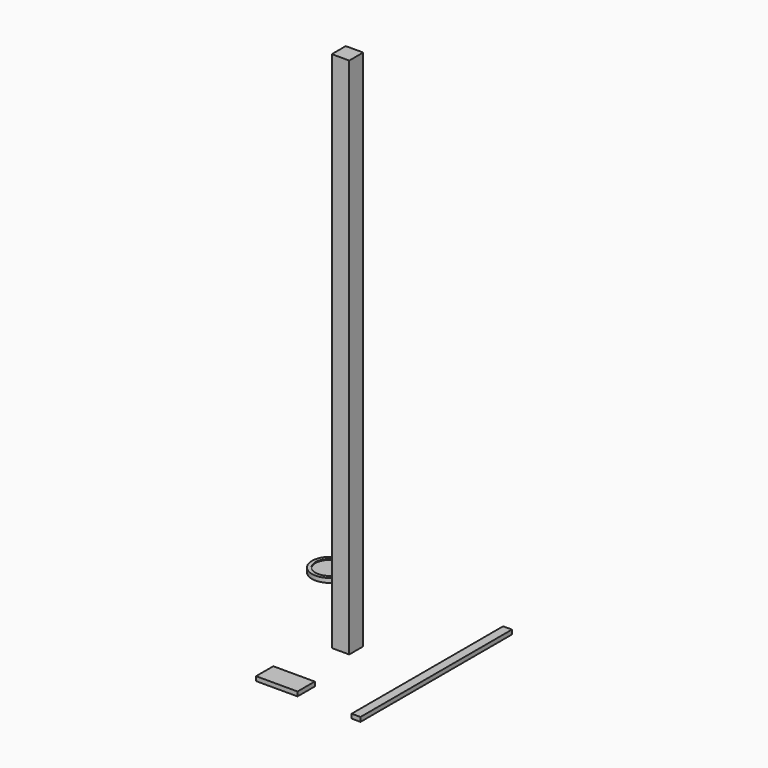
from build123d import *

# Parameters (mm, degrees)
F2_W     = 10.16
F2_H     = 10.16
F3_DEPTH = 304.8
F4_W     = 24.1876728833
F4_H     = 12.5502068549
F5_DEPTH = 2.54
F6_W     = 5.1632523537
F6_H     = 110.3644967079
F7_DEPTH = 2.54
F8_R     = 10.4253047929
F9_DEPTH = 2.54
F11_T    = -2.032


# Not quite as in the source:
# - a feature of the source that left no trace in its solid (it failed there, or was rolled back) is left out


with BuildPart() as f3:
    # F2 (on face) → F3 (new body)
    with BuildSketch(Plane.XY.offset(0.010535121)):
        with Locations((27.4280595768, 76.1781896186)):
            Rectangle(F2_W, F2_H)
    extrude(amount=F3_DEPTH)


with BuildPart() as f5:
    # F4 (on Top) → F5 (new body)
    with BuildSketch(Plane.XY):
        with Locations((27.8465393931, 30.4067051038)):
            Rectangle(F4_W, F4_H)
    extrude(amount=F5_DEPTH)


with BuildPart() as f7:
    # F6 (on Top) → F7 (new body)
    with BuildSketch(Plane.XY):
        with Locations((75.4299908876, 77.6021033525)):
            Rectangle(F6_W, F6_H)
    extrude(amount=F7_DEPTH)


with BuildPart() as f9:
    # F8 (on Top) → F9 (new body)
    with BuildSketch(Plane.XY):
        with Locations((-24.9763578176, 128.8325786591)):
            Circle(F8_R)
    extrude(amount=F9_DEPTH)

    # F11
    f11_openings = [f9.faces().sort_by_distance(p)[0] for p in [
        (-24.976358, 128.832579, 2.54),
    ]]
    offset(amount=F11_T, openings=f11_openings)


solid = Compound([f3.part, f5.part, f7.part, f9.part])
